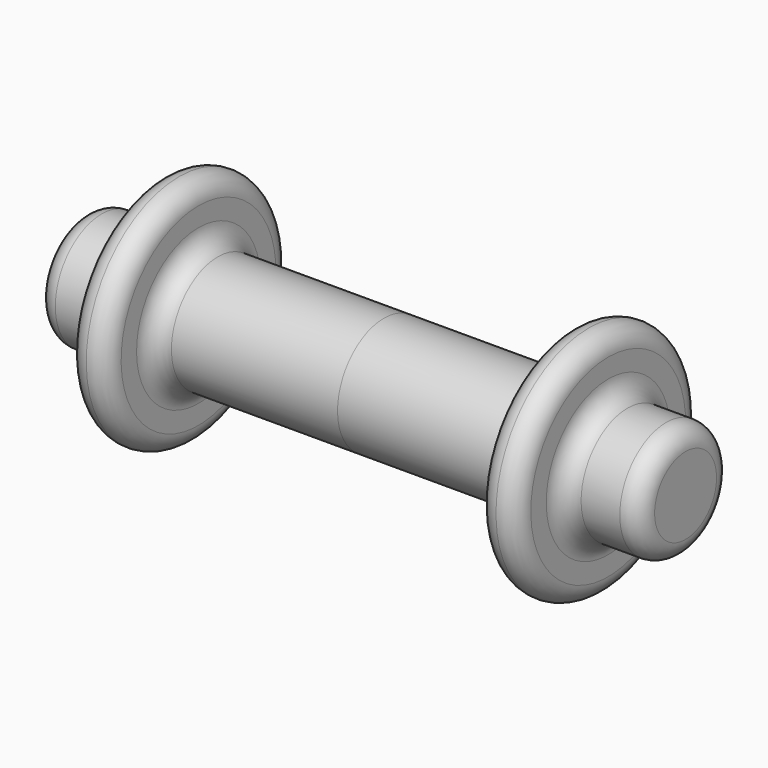
from build123d import *

# Parameters (mm, degrees)
F3_R = 4.99999
F4_R = 5


# Not quite as in the source:
# - a fillet or chamfer is up to 0.001 mm smaller than in the source, because OpenCascade refuses the exact size


with BuildPart() as f1:
    # F0 (on Front) → F1 (revolve)
    with BuildSketch(Plane.XZ):
        with BuildLine():
            Line((0, 15), (0, 0))
            Line((0, 0), (77.9381879678, 0))
            Line((77.9381879678, 0), (77.9381879678, 15))
            Line((77.9381879678, 15), (57.9381879678, 15))
            Line((57.9381879678, 15), (57.9381879678, 30))
            Line((57.9381879678, 30), (47.9381879678, 30))
            Line((47.9381879678, 30), (47.9381879678, 20))
            ThreePointArc((47.9381879678, 20), (46.4737218738, 16.4644660941), (42.9381879678, 15))
            Line((42.9381879678, 15), (0, 15))
        make_face()
    revolve(axis=Axis((38.9690939839, 0, 0), (-1, 0, 0)))

    # F2: F1 across plane


with BuildPart() as f1_1:
    add(f1.part)
    add(f1.part.mirror(Plane.YZ))

    # F3 (radius 5 in the source; OpenCascade refuses exactly that, so slightly less here)
    f3_edges = [f1_1.edges().sort_by_distance(p)[0] for p in [
        (-57.938188, 0, -30),
        (-47.938188, 0, -30),
        (-52.938188, 0, 30),
        (57.938188, 0, -30),
        (47.938188, 0, -30),
        (52.938188, 0, 30),
    ]]
    fillet(f3_edges, radius=F3_R)

    # F4
    f4_edges = [f1_1.edges().sort_by_distance(p)[0] for p in [
        (77.938188, 0, -15),
        (57.938188, 0, -15),
        (67.938188, 0, 15),
        (-77.938188, 0, -15),
        (-57.938188, 0, -15),
        (-67.938188, 0, 15),
    ]]
    fillet(f4_edges, radius=F4_R)


solid = f1_1.part
